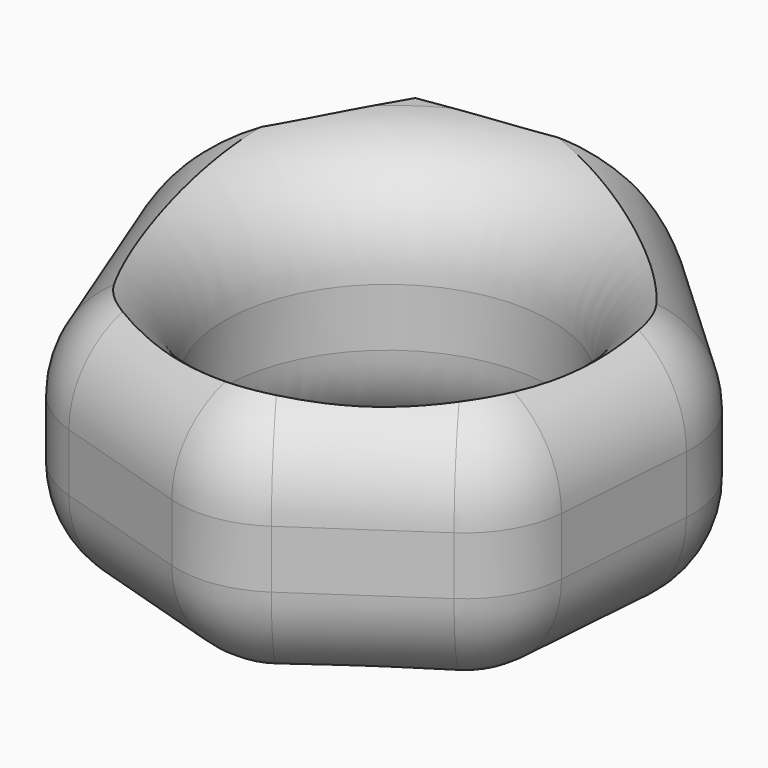
from build123d import *

# Parameters (mm, degrees)
F0_R         = 8
F1_DEPTH     = 13
F2_T1_DEPTH  = 2.84
F2_T3_DEPTH  = 7.0113068008
F2_T5_DEPTH  = 7.0113068008
F2_T7_DEPTH  = 7.0113068008
F2_T9_DEPTH  = 25.2319953177
F2_T11_DEPTH = 22.1577058643
F2_T13_DEPTH = 22.1577058643
F2_T18_DEPTH = 5.08
F2_T24_DEPTH = 5.08
F2_T30_DEPTH = 5.08
F2_T36_DEPTH = 5.08
F2_T42_DEPTH = 5.08
F2_T48_DEPTH = 5.08
F2_T54_DEPTH = 5.08
F2_T60_DEPTH = 5.08


# Not quite as in the source:
# - a fillet or chamfer that OpenCascade refuses, or shapes differently, is made with other operations: its cross-section is extruded or revolved along the edge and cut away or added


with BuildPart() as f1:
    # F0 (on Top) → F1 (new body)
    with BuildSketch(Plane.XY):
        Polygon((-7.71981316, 11.3397637924), (-13.6790091142, 1.0346341127), (-9.3376322044, -10.0495961565), (2.0351722083, -13.5662755455), (11.8754504382, -6.8672727471), (12.7732722731, 5.0029264966), (4.0525595591, 13.1058200473), align=None)
        Circle(F0_R, mode=Mode.SUBTRACT)
    extrude(amount=F1_DEPTH)

    # F2: fillet of radius 5.08 on 19 edges, made by hand

    # F2_s2 → F2_t1 (cut)
    with BuildSketch(Plane.XY.offset(5.08)):
        with BuildLine():
            ThreePointArc((-10.2298236351, -7.7716886015), (-8.9575574192, -9.6405419105), (-7.0004201054, -10.7723049377))
            Line((-7.0004201054, -10.7723049377), (-9.3376322044, -10.0495961565))
            Line((-9.3376322044, -10.0495961565), (-10.2298236351, -7.7716886015))
        make_face()
        with BuildLine():
            ThreePointArc((4.0574365946, -12.1895711001), (1.9523334733, -13.0140799619), (-0.3020398907, -12.8435667642))
            Line((-0.3020398907, -12.8435667642), (2.0351722083, -13.5662755455))
            Line((2.0351722083, -13.5662755455), (4.0574365946, -12.1895711001))
        make_face()
        with BuildLine():
            ThreePointArc((9.8531860519, -8.2439771925), (11.39207744, -6.5877503632), (12.0599607822, -4.4278416022))
            Line((12.0599607822, -4.4278416022), (11.8754504382, -6.8672727471))
            Line((11.8754504382, -6.8672727471), (9.8531860519, -8.2439771925))
        make_face()
        with BuildLine():
            ThreePointArc((12.588761929, 2.5634953517), (12.2533547384, 4.7992896247), (10.9810885225, 6.6681429337))
            Line((10.9810885225, 6.6681429337), (12.7732722731, 5.0029264966))
            Line((12.7732722731, 5.0029264966), (12.588761929, 2.5634953517))
        make_face()
    extrude(amount=F2_T1_DEPTH, mode=Mode.SUBTRACT)

    # F2_s4 → F2_t3 (cut)
    with BuildSketch(Plane(origin=(-3.3491901073, 1.0356309133, 0), x_dir=(0, 0, 1), z_dir=(0.9553682937, -0.2954173716, 0))):
        with BuildLine():
            ThreePointArc((5.08, 12.3595642949), (1.4878975516, 10.8716667433), (0, 7.2795642949))
            Line((0, 7.2795642949), (0, 12.3595642949))
            Line((0, 12.3595642949), (5.08, 12.3595642949))
        make_face()
        with BuildLine():
            ThreePointArc((7.92, 12.3595642949), (11.5121024484, 10.8716667433), (13, 7.2795642949))
            Line((13, 7.2795642949), (13, 12.3595642949))
            Line((13, 12.3595642949), (7.92, 12.3595642949))
        make_face()
    extrude(amount=F2_T3_DEPTH, mode=Mode.SUBTRACT)

    # F2_s6 → F2_t5 (cut)
    with BuildSketch(Plane(origin=(-2.8978747286, -1.9727969538, 0), x_dir=(0, 0, 1), z_dir=(0.8266289897, 0.5627472909, 0))):
        with BuildLine():
            ThreePointArc((5.08, 12.3595642949), (1.4878975516, 10.8716667433), (0, 7.2795642949))
            Line((0, 7.2795642949), (0, 12.3595642949))
            Line((0, 12.3595642949), (5.08, 12.3595642949))
        make_face()
        with BuildLine():
            ThreePointArc((7.92, 12.3595642949), (11.5121024484, 10.8716667433), (13, 7.2795642949))
            Line((13, 7.2795642949), (13, 12.3595642949))
            Line((13, 12.3595642949), (7.92, 12.3595642949))
        make_face()
    extrude(amount=F2_T5_DEPTH, mode=Mode.SUBTRACT)

    # F2_s8 → F2_t7 (cut)
    with BuildSketch(Plane(origin=(-0.2644005734, -3.4956684769, 0), x_dir=(0, 0, 1), z_dir=(0.0754211963, 0.9971517654, 0))):
        with BuildLine():
            ThreePointArc((5.08, 12.3595642949), (1.4878975516, 10.8716667433), (0, 7.2795642949))
            Line((0, 7.2795642949), (0, 12.3595642949))
            Line((0, 12.3595642949), (5.08, 12.3595642949))
        make_face()
        with BuildLine():
            ThreePointArc((7.92, 12.3595642949), (11.5121024484, 10.8716667433), (13, 7.2795642949))
            Line((13, 7.2795642949), (13, 12.3595642949))
            Line((13, 12.3595642949), (7.92, 12.3595642949))
        make_face()
    extrude(amount=F2_T7_DEPTH, mode=Mode.SUBTRACT)

    # F2_s10 → F2_t9 (cut)
    with BuildSketch(Plane.XY.offset(-6.1159976589)):
        with BuildLine():
            ThreePointArc((-12.4543415319, 3.1524295918), (-13.1222248741, 0.9925208307), (-12.7868176835, -1.2432734423))
            Line((-12.7868176835, -1.2432734423), (-13.6790091142, 1.0346341127))
            Line((-13.6790091142, 1.0346341127), (-12.4543415319, 3.1524295918))
        make_face()
        with BuildLine():
            ThreePointArc((5.8447433097, 11.4406036103), (3.8876059959, 12.5723666375), (1.6332326319, 12.7428798351))
            Line((1.6332326319, 12.7428798351), (4.0525595591, 13.1058200473))
            Line((4.0525595591, 13.1058200473), (5.8447433097, 11.4406036103))
        make_face()
    extrude(amount=F2_T9_DEPTH, mode=Mode.SUBTRACT)

    # F2_s12 → F2_t11 (cut)
    with BuildSketch(Plane(origin=(-6.802324944, 17.367424578, 0), x_dir=(0, 0, 1), z_dir=(0.3646957865, -0.9311267278, 0))):
        with BuildLine():
            ThreePointArc((5.08, 12.3595642949), (1.4878975516, 10.8716667433), (0, 7.2795642949))
            Line((0, 7.2795642949), (0, 12.3595642949))
            Line((0, 12.3595642949), (5.08, 12.3595642949))
        make_face()
        with BuildLine():
            ThreePointArc((7.92, 12.3595642949), (11.5121024484, 10.8716667433), (13, 7.2795642949))
            Line((13, 7.2795642949), (13, 12.3595642949))
            Line((13, 12.3595642949), (7.92, 12.3595642949))
        make_face()
    extrude(amount=F2_T11_DEPTH, mode=Mode.SUBTRACT)

    # F2_s14 → F2_t13 (cut)
    with BuildSketch(Plane(origin=(2.5681726064, -2.3862303383, 0), x_dir=(0, 0, 1), z_dir=(-0.7325802962, 0.6806806223, 0))):
        with BuildLine():
            ThreePointArc((5.08, 12.3595642949), (1.4878975516, 10.8716667433), (0, 7.2795642949))
            Line((0, 7.2795642949), (0, 12.3595642949))
            Line((0, 12.3595642949), (5.08, 12.3595642949))
        make_face()
        with BuildLine():
            ThreePointArc((7.92, 12.3595642949), (11.5121024484, 10.8716667433), (13, 7.2795642949))
            Line((13, 7.2795642949), (13, 12.3595642949))
            Line((13, 12.3595642949), (7.92, 12.3595642949))
        make_face()
    extrude(amount=F2_T13_DEPTH, mode=Mode.SUBTRACT)


with BuildPart() as f2_tool16:
    # F2_s17 → F2_t18 (new body)
    with BuildSketch(Plane.XY.offset(5.08)):
        Polygon((-5.4996998577, -5.9190340058), (-10.2298236351, -7.7716886015), (-9.3376322044, -10.0495961565), (-7.0004201054, -10.7723049377), align=None)
    extrude(amount=-F2_T18_DEPTH)

    # F2_s19 → F2_t20 (revolve, cut)
    with BuildSketch(Plane(origin=(-5.4996998577, -5.9190340058, 5.08), x_dir=(0.6806806223, 0.7325802962, 0), z_dir=(-0.7325802962, 0.6806806223, 0))):
        with BuildLine():
            ThreePointArc((0, -5.08), (5.08, 0), (0, 5.08))
            Line((0, 5.08), (0, -5.08))
        make_face()
    revolve(axis=Axis((-5.4996998577, -5.9190340058, 5.08), (0, 0, -1)), mode=Mode.SUBTRACT)


with BuildPart() as f1_1:
    add(f1.part)

    # F2_t15: cut F2_tool16
    add(f2_tool16.part, mode=Mode.SUBTRACT)


with BuildPart() as f2_tool22:
    # F2_s23 → F2_t24 (new body)
    with BuildSketch(Plane.XY.offset(7.92)):
        Polygon((-5.4996998577, -5.9190340058), (-10.2298236351, -7.7716886015), (-9.3376322044, -10.0495961565), (-7.0004201054, -10.7723049377), align=None)
    extrude(amount=F2_T24_DEPTH)

    # F2_s25 → F2_t26 (revolve, cut)
    with BuildSketch(Plane(origin=(-5.4996998577, -5.9190340058, 7.92), x_dir=(0.6806806223, 0.7325802962, 0), z_dir=(0.7325802962, -0.6806806223, 0))):
        with BuildLine():
            ThreePointArc((0, -5.08), (5.08, 0), (0, 5.08))
            Line((0, 5.08), (0, -5.08))
        make_face()
    revolve(axis=Axis((-5.4996998577, -5.9190340058, 7.92), (0, 0, 1)), mode=Mode.SUBTRACT)


with BuildPart() as f1_2:
    add(f1_1.part)

    # F2_t21: cut F2_tool22
    add(f2_tool22.part, mode=Mode.SUBTRACT)


with BuildPart() as f2_tool28:
    # F2_s29 → F2_t30 (new body)
    with BuildSketch(Plane.XY.offset(5.08)):
        Polygon((1.198680357, -7.9902958324), (-0.3020398907, -12.8435667642), (2.0351722083, -13.5662755455), (4.0574365946, -12.1895711001), align=None)
    extrude(amount=-F2_T30_DEPTH)

    # F2_s31 → F2_t32 (revolve, cut)
    with BuildSketch(Plane(origin=(1.198680357, -7.9902958324, 5.08), x_dir=(-0.1483569126, 0.9889338838, 0), z_dir=(-0.9889338838, -0.1483569126, 0))):
        with BuildLine():
            ThreePointArc((0, -5.08), (5.08, 0), (0, 5.08))
            Line((0, 5.08), (0, -5.08))
        make_face()
    revolve(axis=Axis((1.198680357, -7.9902958324, 5.08), (0, 0, -1)), mode=Mode.SUBTRACT)


with BuildPart() as f1_3:
    add(f1_2.part)

    # F2_t27: cut F2_tool28
    add(f2_tool28.part, mode=Mode.SUBTRACT)


with BuildPart() as f2_tool34:
    # F2_s35 → F2_t36 (new body)
    with BuildSketch(Plane.XY.offset(7.92)):
        Polygon((1.198680357, -7.9902958324), (-0.3020398907, -12.8435667642), (2.0351722083, -13.5662755455), (4.0574365946, -12.1895711001), align=None)
    extrude(amount=F2_T36_DEPTH)

    # F2_s37 → F2_t38 (revolve, cut)
    with BuildSketch(Plane(origin=(1.198680357, -7.9902958324, 7.92), x_dir=(-0.1483569126, 0.9889338838, 0), z_dir=(0.9889338838, 0.1483569126, 0))):
        with BuildLine():
            ThreePointArc((0, -5.08), (5.08, 0), (0, 5.08))
            Line((0, 5.08), (0, -5.08))
        make_face()
    revolve(axis=Axis((1.198680357, -7.9902958324, 7.92), (0, 0, 1)), mode=Mode.SUBTRACT)


with BuildPart() as f1_4:
    add(f1_3.part)

    # F2_t33: cut F2_tool34
    add(f2_tool34.part, mode=Mode.SUBTRACT)


with BuildPart() as f2_tool40:
    # F2_s41 → F2_t42 (new body)
    with BuildSketch(Plane.XY.offset(5.08)):
        Polygon((6.9944298143, -4.0447019248), (9.8531860519, -8.2439771925), (11.8754504382, -6.8672727471), (12.0599607822, -4.4278416022), align=None)
    extrude(amount=-F2_T42_DEPTH)

    # F2_s43 → F2_t44 (revolve, cut)
    with BuildSketch(Plane(origin=(6.9944298143, -4.0447019248, 5.08), x_dir=(-0.8656786665, 0.5006000863, 0), z_dir=(-0.5006000863, -0.8656786665, 0))):
        with BuildLine():
            ThreePointArc((0, -5.08), (5.08, 0), (0, 5.08))
            Line((0, 5.08), (0, -5.08))
        make_face()
    revolve(axis=Axis((6.9944298143, -4.0447019248, 5.08), (0, 0, -1)), mode=Mode.SUBTRACT)


with BuildPart() as f1_5:
    add(f1_4.part)

    # F2_t39: cut F2_tool40
    add(f2_tool40.part, mode=Mode.SUBTRACT)


with BuildPart() as f2_tool46:
    # F2_s47 → F2_t48 (new body)
    with BuildSketch(Plane.XY.offset(7.92)):
        Polygon((6.9944298143, -4.0447019248), (9.8531860519, -8.2439771925), (11.8754504382, -6.8672727471), (12.0599607822, -4.4278416022), align=None)
    extrude(amount=F2_T48_DEPTH)

    # F2_s49 → F2_t50 (revolve, cut)
    with BuildSketch(Plane(origin=(6.9944298143, -4.0447019248, 7.92), x_dir=(-0.8656786665, 0.5006000863, 0), z_dir=(0.5006000863, 0.8656786665, 0))):
        with BuildLine():
            ThreePointArc((0, -5.08), (5.08, 0), (0, 5.08))
            Line((0, 5.08), (0, -5.08))
        make_face()
    revolve(axis=Axis((6.9944298143, -4.0447019248, 7.92), (0, 0, 1)), mode=Mode.SUBTRACT)


with BuildPart() as f1_6:
    add(f1_5.part)

    # F2_t45: cut F2_tool46
    add(f2_tool46.part, mode=Mode.SUBTRACT)


with BuildPart() as f2_tool52:
    # F2_s53 → F2_t54 (new body)
    with BuildSketch(Plane.XY.offset(5.08)):
        Polygon((7.523230961, 2.946635029), (12.588761929, 2.5634953517), (12.7732722731, 5.0029264966), (10.9810885225, 6.6681429337), align=None)
    extrude(amount=-F2_T54_DEPTH)

    # F2_s55 → F2_t56 (revolve, cut)
    with BuildSketch(Plane(origin=(7.523230961, 2.946635029, 5.08), x_dir=(-0.9311267278, -0.3646957865, 0), z_dir=(0.3646957865, -0.9311267278, 0))):
        with BuildLine():
            ThreePointArc((0, -5.08), (5.08, 0), (0, 5.08))
            Line((0, 5.08), (0, -5.08))
        make_face()
    revolve(axis=Axis((7.523230961, 2.946635029, 5.08), (0, 0, -1)), mode=Mode.SUBTRACT)


with BuildPart() as f1_7:
    add(f1_6.part)

    # F2_t51: cut F2_tool52
    add(f2_tool52.part, mode=Mode.SUBTRACT)


with BuildPart() as f2_tool58:
    # F2_s59 → F2_t60 (new body)
    with BuildSketch(Plane.XY.offset(7.92)):
        Polygon((7.523230961, 2.946635029), (12.588761929, 2.5634953517), (12.7732722731, 5.0029264966), (10.9810885225, 6.6681429337), align=None)
    extrude(amount=F2_T60_DEPTH)

    # F2_s61 → F2_t62 (revolve, cut)
    with BuildSketch(Plane(origin=(7.523230961, 2.946635029, 7.92), x_dir=(-0.9311267278, -0.3646957865, 0), z_dir=(-0.3646957865, 0.9311267278, 0))):
        with BuildLine():
            ThreePointArc((0, -5.08), (5.08, 0), (0, 5.08))
            Line((0, 5.08), (0, -5.08))
        make_face()
    revolve(axis=Axis((7.523230961, 2.946635029, 7.92), (0, 0, 1)), mode=Mode.SUBTRACT)


with BuildPart() as f1_8:
    add(f1_7.part)

    # F2_t57: cut F2_tool58
    add(f2_tool58.part, mode=Mode.SUBTRACT)

    # F2_s63 → F2_t64 (revolve, cut)
    with BuildSketch(Plane.XZ):
        with BuildLine():
            ThreePointArc((8, 5.08), (9.4878975516, 1.4878975516), (13.08, 0))
            Line((13.08, 0), (8, 0))
            Line((8, 0), (8, 5.08))
        make_face()
    revolve(axis=Axis((0, 0, 0), (0, 0, 1)), mode=Mode.SUBTRACT)

    # F2_s65 → F2_t66 (revolve, cut)
    with BuildSketch(Plane.XZ):
        with BuildLine():
            ThreePointArc((8, 7.92), (9.4878975516, 11.5121024484), (13.08, 13))
            Line((13.08, 13), (8, 13))
            Line((8, 13), (8, 7.92))
        make_face()
    revolve(axis=Axis((0, 0, 13), (0, 0, 1)), mode=Mode.SUBTRACT)


solid = f1_8.part
